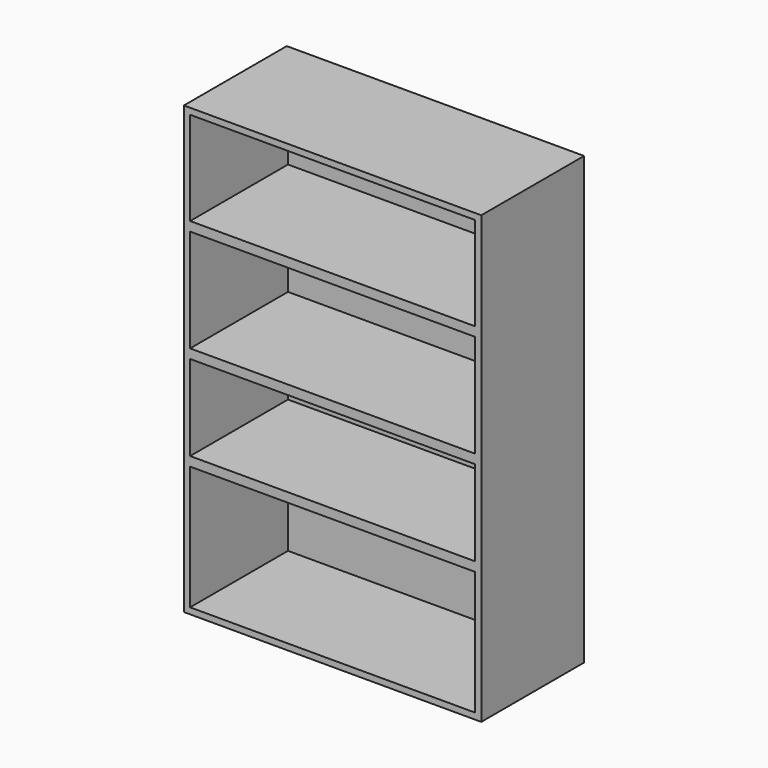
from build123d import *

# Parameters (mm, degrees)
F0_W     = 609.6
F0_H     = 914.4
F1_DEPTH = 263.525
F2_T     = -12.7
F3_W     = 584.2
F3_H     = 19.05
F4_DEPTH = 250.825
F5_W     = 584.2
F5_H     = 19.05
F6_DEPTH = 250.825


# Not quite as in the source:
# - the program builds the solid bodies; features that only make, move or delete a surface that nothing else refers to are left out


with BuildPart() as f1:
    # F0 (on Front) → F1 (new body)
    with BuildSketch(Plane.XZ):
        Rectangle(F0_W, F0_H)
    extrude(amount=F1_DEPTH)

    # F2
    f2_openings = [f1.faces().sort_by_distance(p)[0] for p in [
        (0, -263.525, 0),
    ]]
    offset(amount=F2_T, openings=f2_openings)

    # F3 (on face) → F4 (join)
    with BuildSketch(Plane.XZ.offset(12.7)):
        with Locations((0, -180.975)):
            Rectangle(F3_W, F3_H)
    extrude(amount=F4_DEPTH)

    # F5 (on face) → F6 (join)
    with BuildSketch(Plane.XZ.offset(12.7)):
        with Locations((0, 13.335)):
            Rectangle(F5_W, F5_H)
        with Locations((0, 243.205)):
            Rectangle(F5_W, F5_H)
    extrude(amount=F6_DEPTH)


solid = f1.part
